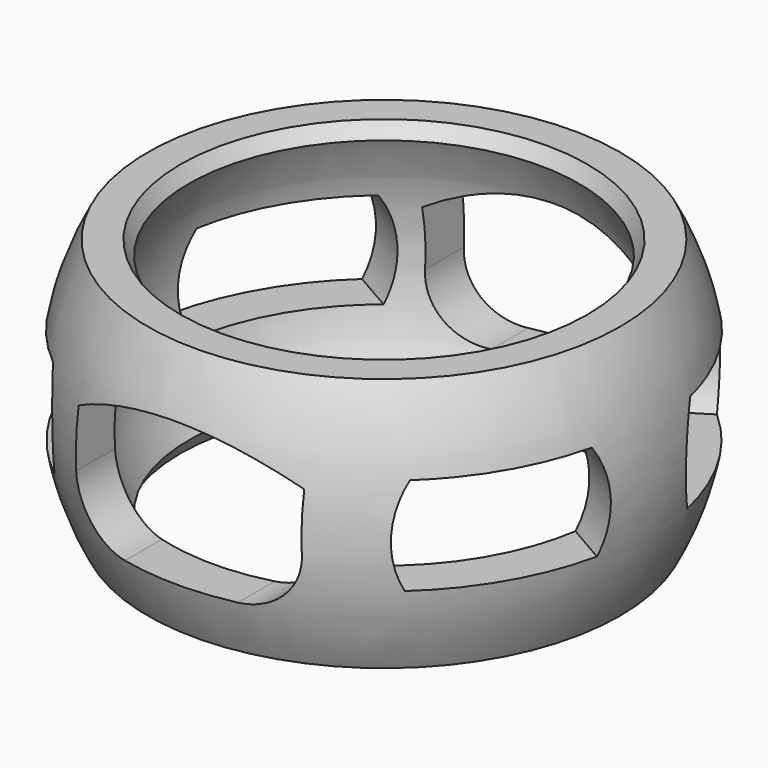
from build123d import *

# Parameters (mm, degrees)
F6_DEPTH  = 38.1
F11_DEPTH = 76.2
F13_DEPTH = 76.2


# Not quite as in the source:
# - a fillet or chamfer that OpenCascade refuses, or shapes differently, is made with other operations: its cross-section is extruded or revolved along the edge and cut away or added


with BuildPart() as f2:
    # F0 (on Front) → F2 (revolve)
    with BuildSketch(Plane.XZ):
        with BuildLine():
            Line((21.0006510316, -14.2875), (26.611533725, -14.2875))
            ThreePointArc((26.611533725, -14.2875), (30.20441, 0), (26.611533725, 14.2875))
            Line((26.611533725, 14.2875), (21.0006510316, 14.2875))
            ThreePointArc((21.0006510316, 14.2875), (25.4, 0), (21.0006510316, -14.2875))
        make_face()
    revolve(axis=Axis((0.0936897777, 0, 16.2081146991), (0, 0, 1)))

    # F3: chamfer of 2.032 on 2 edges, made by hand

    # F3_s1 → F3_t2 (revolve, cut)
    with BuildSketch(Plane.XZ):
        with BuildLine():
            Line((22.9835206872, 14.357868075), (21.9703898741, 12.6053114603))
            Line((21.9703898741, 12.6053114603), (21.9351721641, 12.585030373))
            ThreePointArc((21.9351721641, 12.585030373), (21.496616359, 13.4533499443), (20.9670499899, 14.26464))
            Line((20.9670499899, 14.26464), (21.0006510316, 14.32814))
            ThreePointArc((21.0006510316, 14.32814), (21.9920858594, 14.32814), (22.9835206872, 14.398508075))
            Line((22.9835206872, 14.398508075), (22.9835206872, 14.357868075))
        make_face()
    revolve(axis=Axis((0.0936897777, 0, 14.2875), (0, 0, 1)), mode=Mode.SUBTRACT)

    # F3_s3 → F3_t4 (revolve, cut)
    with BuildSketch(Plane.XZ):
        with BuildLine():
            Line((22.9835206872, -14.357868075), (21.9703898741, -12.6053114603))
            Line((21.9703898741, -12.6053114603), (21.9351721641, -12.585030373))
            ThreePointArc((21.9351721641, -12.585030373), (21.496616359, -13.4533499443), (20.9670499899, -14.26464))
            Line((20.9670499899, -14.26464), (21.0006510316, -14.32814))
            ThreePointArc((21.0006510316, -14.32814), (21.9920858594, -14.32814), (22.9835206872, -14.398508075))
            Line((22.9835206872, -14.398508075), (22.9835206872, -14.357868075))
        make_face()
    revolve(axis=Axis((0.0936897777, 0, -14.2875), (0, 0, 1)), mode=Mode.SUBTRACT)

    # F5 (on Front) → F6 (cut, symmetric)
    with BuildSketch(Plane.XZ):
        with BuildLine():
            ThreePointArc((6.35, -8.0514773719), (1.8598719395, -6.1916054325), (0, -1.7014773719))
            Line((0, -1.7014773719), (0, -8.0514773719))
            Line((0, -8.0514773719), (6.35, -8.0514773719))
        make_face()
        with BuildLine():
            Line((0, -8.0514773719), (0, -1.7014773719))
            ThreePointArc((0, -1.7014773719), (-1.8598719395, -6.1916054325), (-6.35, -8.0514773719))
            Line((-6.35, -8.0514773719), (0, -8.0514773719))
        make_face()
        with BuildLine():
            ThreePointArc((0.2322001706, 0), (0.0583178356, -0.8428531575), (0, -1.7014773719))
            ThreePointArc((0, -1.7014773719), (1.8598719395, -6.1916054325), (6.35, -8.0514773719))
            ThreePointArc((6.35, -8.0514773719), (10.8401280605, -6.1916054325), (12.7, -1.7014773719))
            ThreePointArc((12.7, -1.7014773719), (10.8401280588, 2.7886506904), (6.349999995, 4.6485226281))
            ThreePointArc((6.349999995, 4.6485226281), (2.508247879, 3.3545527546), (0.2322001706, 0))
        make_face()
        with BuildLine():
            ThreePointArc((0, -1.7014773719), (-1.8598719395, 2.7886506886), (-6.35, 4.6485226281))
            ThreePointArc((-6.35, 4.6485226281), (-10.8401280605, 2.7886506886), (-12.7, -1.7014773719))
            ThreePointArc((-12.7, -1.7014773719), (-10.8401280605, -6.1916054325), (-6.35, -8.0514773719))
            ThreePointArc((-6.35, -8.0514773719), (-1.8598719395, -6.1916054325), (0, -1.7014773719))
        make_face()
        with BuildLine():
            Line((12.7, -1.7014773719), (12.7, 4.6485226281))
            Line((12.7, 4.6485226281), (6.349999995, 4.6485226281))
            ThreePointArc((6.349999995, 4.6485226281), (10.8401280588, 2.7886506904), (12.7, -1.7014773719))
        make_face()
        with BuildLine():
            Line((-6.35, 4.6485226281), (-12.7, 4.6485226281))
            Line((-12.7, 4.6485226281), (-12.7, -1.7014773719))
            ThreePointArc((-12.7, -1.7014773719), (-10.8401280605, 2.7886506886), (-6.35, 4.6485226281))
        make_face()
        with BuildLine():
            Line((6.349999995, 4.6485226281), (0, 4.6485226281))
            Line((0, 4.6485226281), (0, 0))
            Line((0, 0), (0.2322001706, 0))
            ThreePointArc((0.2322001706, 0), (2.508247879, 3.3545527546), (6.349999995, 4.6485226281))
        make_face()
        with BuildLine():
            ThreePointArc((12.7, 4.6485226281), (6.5740037456, 7.1859933597), (0, 8.0514773719))
            Line((0, 8.0514773719), (0, 4.6485226281))
            Line((0, 4.6485226281), (6.349999995, 4.6485226281))
            Line((6.349999995, 4.6485226281), (12.7, 4.6485226281))
        make_face()
        with BuildLine():
            Line((0, 4.6485226281), (-6.35, 4.6485226281))
            ThreePointArc((-6.35, 4.6485226281), (-1.8598719395, 2.7886506886), (0, -1.7014773719))
            Line((0, -1.7014773719), (0, 0))
            Line((0, 0), (0, 4.6485226281))
        make_face()
        with BuildLine():
            ThreePointArc((0, 8.0514773719), (-6.5740037456, 7.1859933597), (-12.7, 4.6485226281))
            Line((-12.7, 4.6485226281), (-6.35, 4.6485226281))
            Line((-6.35, 4.6485226281), (0, 4.6485226281))
            Line((0, 4.6485226281), (0, 8.0514773719))
        make_face()
        with BuildLine():
            Line((0, 0), (0, -1.7014773719))
            ThreePointArc((0, -1.7014773719), (0.0583178356, -0.8428531575), (0.2322001706, 0))
            Line((0.2322001706, 0), (0, 0))
        make_face()
    extrude(amount=F6_DEPTH, both=True, mode=Mode.SUBTRACT)

    # F10 (on line) → F11 (cut)
    with BuildSketch(Plane(origin=(-26.1544868095, 15.1003, 0), x_dir=(0.5, 0.8660254038, 0), z_dir=(0.8660254038, -0.5, 0))):
        with BuildLine():
            Line((8.5551824144, 5.8214371093), (-8.5551824144, 5.8214371093))
            ThreePointArc((-8.5551824144, 5.8214371093), (-10.3378059029, 0.4583069663), (-9.0367714612, -5.0415312871))
            Line((-9.0367714612, -5.0415312871), (0, -5.0415312871))
            Line((0, -5.0415312871), (9.0367714612, -5.0415312871))
            ThreePointArc((9.0367714612, -5.0415312871), (10.3378059029, 0.4583069663), (8.5551824144, 5.8214371093))
        make_face()
    extrude(amount=F11_DEPTH, mode=Mode.SUBTRACT)

    # F12 (on face) → F13 (cut)
    with BuildSketch(Plane(origin=(-25.6163563103, -16.0033956657, 0), x_dir=(-0.5298363936, 0.8480998738, 0), z_dir=(0.8480998738, 0.5298363936, 0))):
        with BuildLine():
            Line((7.7066458478, 5.3130234251), (-9.4037189811, 5.3130234251))
            ThreePointArc((-9.4037189811, 5.3130234251), (-11.1863424695, -0.0501067179), (-9.8853080279, -5.5499449713))
            Line((-9.8853080279, -5.5499449713), (-0.8485365666, -5.5499449713))
            Line((-0.8485365666, -5.5499449713), (8.1882348946, -5.5499449713))
            ThreePointArc((8.1882348946, -5.5499449713), (9.4892693363, -0.0501067179), (7.7066458478, 5.3130234251))
        make_face()
    extrude(amount=F13_DEPTH, mode=Mode.SUBTRACT)


solid = f2.part
